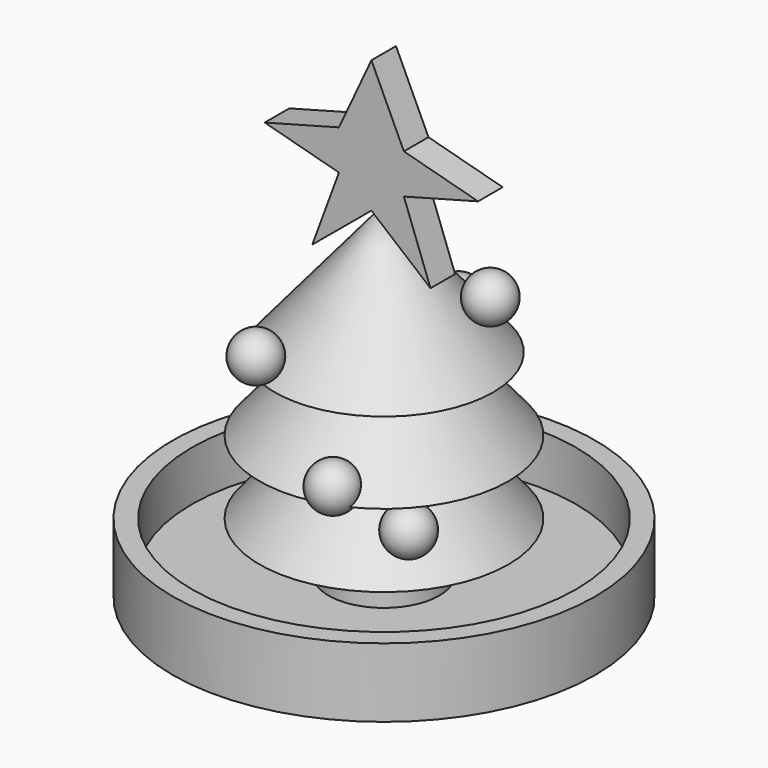
from build123d import *

# Parameters (mm, degrees)
F0_W          = 9.1577712446
F0_H          = 11.4250707794
F3_R          = 34.925
F3_R_2        = 31.75
F4_DEPTH      = 11.43
F3_R_3        = 9.1577712446
F5_DEPTH      = 3.175
F7_DEPTH      = 2.54
F7_DEPTH_BACK = 2.54


with BuildPart() as f1:
    # F0 (on Front) → F1 (revolve)
    with BuildSketch(Plane.XZ):
        Polygon((0, 38.593464756), (0, -7.1314644646), (9.1577712446, -7.1314644646), (20.5877712446, -7.1314644646), (10.4277712446, 4.9767520361), (20.5877712446, 4.9767520361), (10.4277712446, 17.0849685369), (18.0477712446, 17.0849685369), align=None)
    revolve(axis=Axis((0, 0, 3.668464756), (0, 0, 1)))

    # F20 (on offset) → F21 (revolve)
    with BuildSketch(Plane.YZ.offset(-16.51)):
        with BuildLine():
            Line((5.9082479449, 11.1316262284), (5.9082479449, 18.7516262284))
            ThreePointArc((5.9082479449, 18.7516262284), (2.0982479449, 14.9416262284), (5.9082479449, 11.1316262284))
        make_face()
    revolve(axis=Axis((-16.51, 5.9082479449, 14.9416262284), (0, 0, -1)))


with BuildPart() as f2:
    # F0 (on Front) → F2 (revolve)
    with BuildSketch(Plane.XZ):
        with Locations((4.5788856223, -12.8439998543)):
            Rectangle(F0_W, F0_H)
    revolve(axis=Axis((0, 0, 3.668464756), (0, 0, 1)))


with BuildPart() as f4:
    # F3 (on face) → F4 (new body)
    with BuildSketch(Plane(origin=(0, 0, -18.556535244), x_dir=(1, 0, 0), z_dir=(0, 0, -1))):
        Circle(F3_R)
        Circle(F3_R_2, mode=Mode.SUBTRACT)
    extrude(amount=-F4_DEPTH)


with BuildPart() as f5:
    # F3 (on face) → F5 (new body)
    with BuildSketch(Plane(origin=(0, 0, -18.556535244), x_dir=(1, 0, 0), z_dir=(0, 0, -1))):
        Circle(F3_R_2)
        Circle(F3_R_3, mode=Mode.SUBTRACT)
    extrude(amount=-F5_DEPTH)


with BuildPart() as f7:
    # F6 (on Front) → F7 (new body, two sides)
    with BuildSketch(Plane.XZ) as f7_sk:
        Polygon((5.3197673585, 49.0486283282), (-0.0474845656, 60.5587372235), (-5.4147364897, 49.0486283282), (-17.6819944836, 45.7616264554), (-5.4147364897, 42.4746245826), (-9.8146697935, 30.5611621588), (-0.0474845656, 38.6785566129), (9.7197006624, 30.5611621588), (5.3197673585, 42.4746245826), (17.5870253524, 45.7616264554), align=None)
    extrude(amount=-F7_DEPTH)
    extrude(f7_sk.sketch, amount=F7_DEPTH_BACK)


with BuildPart() as f10:
    # F9 (on offset) → F10 (revolve)
    with BuildSketch(Plane.XZ.offset(17.78)):
        with BuildLine():
            Line((-6.9599994458, 17.6474247128), (-6.9599994458, 25.2674247128))
            ThreePointArc((-6.9599994458, 25.2674247128), (-10.7699994458, 21.4574247128), (-6.9599994458, 17.6474247128))
        make_face()
    revolve(axis=Axis((-6.9599994458, -17.78, 21.4574247128), (0, 0, -1)))


with BuildPart() as f11:
    # F9 (on offset) → F11 (revolve)
    with BuildSketch(Plane.XZ.offset(17.78)):
        with BuildLine():
            Line((5.7716159383, 2.8338727081), (5.7716159383, 10.4538727081))
            ThreePointArc((5.7716159383, 10.4538727081), (1.9616159383, 6.6438727081), (5.7716159383, 2.8338727081))
        make_face()
    revolve(axis=Axis((5.7716159383, -17.78, 6.6438727081), (0, 0, -1)))


with BuildPart() as f14:
    # F13 (on offset) → F14 (revolve)
    with BuildSketch(Plane.YZ.offset(13.716)):
        with BuildLine():
            Line((4.8140496248, 23.7740945542), (4.8140496248, 31.3940945542))
            ThreePointArc((4.8140496248, 31.3940945542), (1.0040496248, 27.5840945542), (4.8140496248, 23.7740945542))
        make_face()
    revolve(axis=Axis((13.716, 4.8140496248, 27.5840945542), (0, 0, -1)))


with BuildPart() as f15:
    # F13 (on offset) → F15 (revolve)
    with BuildSketch(Plane.YZ.offset(13.716)):
        with BuildLine():
            Line((-12.0565985097, -3.2672330271), (-12.0565985097, 4.3527669729))
            ThreePointArc((-12.0565985097, 4.3527669729), (-15.8665985097, 0.5427669729), (-12.0565985097, -3.2672330271))
        make_face()
    revolve(axis=Axis((13.716, -12.0565985097, 0.5427669729), (0, 0, -1)))


with BuildPart() as f18:
    # F17 (on offset) → F18 (revolve)
    with BuildSketch(Plane.XZ.offset(-18.288)):
        with BuildLine():
            Line((-2.2855464602, 12.5775911385), (-2.2855464602, 20.1975911385))
            ThreePointArc((-2.2855464602, 20.1975911385), (-6.0955464602, 16.3875911385), (-2.2855464602, 12.5775911385))
        make_face()
    revolve(axis=Axis((-2.2855464602, 18.288, 16.3875911385), (0, 0, -1)))


with BuildPart() as f22:
    # F20 (on offset) → F22 (revolve)
    with BuildSketch(Plane.YZ.offset(-16.51)):
        with BuildLine():
            Line((13.6200552108, -7.6199638129), (13.6366607621, 0))
            ThreePointArc((13.6366607621, 0), (9.8100642575, -3.8016610175), (13.6200552108, -7.6199638129))
        make_face()
    revolve(axis=Axis((-16.51, 13.6283579864, -3.8099819065), (0, -0.0021792114, -0.9999976255)))


solid = Compound([f1.part, f2.part, f4.part, f5.part, f7.part, f10.part, f11.part, f14.part, f15.part, f18.part, f22.part])
